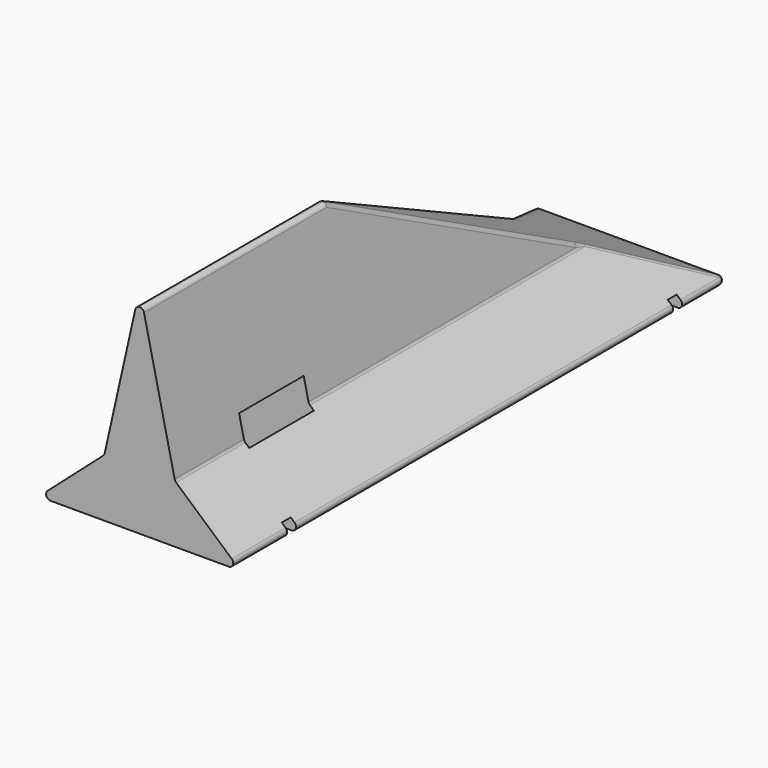
from build123d import *

# Parameters (mm, degrees)
F1_DEPTH = 28.575
F3_DEPTH = 22.86
F5_DEPTH = 177.8
F6_R     = 1.27


with BuildPart() as f1:
    # F0 (on Right) → F1 (new body, symmetric)
    with BuildSketch(Plane.YZ):
        Polygon((-57.9421781003, 88.9), (-57.9421781003, 0), (-38.8921781003, 0), (-38.8921781003, 3.175), (-35.7171781003, 3.175), (-35.7171781003, 0), (97.6328218997, 0), (97.6328218997, 3.175), (100.8078218997, 3.175), (100.8078218997, 0), (119.8578218997, 0), align=None)
    extrude(amount=F1_DEPTH, both=True)

    # F2 (on face) → F3 (cut)
    with BuildSketch(Plane(origin=(0, 0, 0), x_dir=(1, 0, 0), z_dir=(0, 0, -1))):
        Polygon((11.43, 33.4499907649), (0, 33.4499907649), (-11.43, 33.4499907649), (-11.43, 10.5899907649), (0, 10.5899907649), (11.43, 10.5899907649), align=None)
    extrude(amount=-F3_DEPTH, mode=Mode.SUBTRACT)

    # F4 (on face) → F5 (intersect)
    with BuildSketch(Plane.XZ.offset(57.9421781003)):
        Polygon((-9.9975576818, 16.3837641232), (-28.575, 0), (28.575, 0), (9.9975576818, 16.3837641232), (0, 60.9972961555), align=None)
    extrude(amount=-F5_DEPTH, mode=Mode.INTERSECT)

    # F6
    f6_edges = [f1.edges().sort_by_distance(p)[0] for p in [
        (0, 119.857822, 0),
        (4.998779, 42.476762, 38.69053),
        (-4.998779, 42.476762, 38.69053),
        (19.286279, 103.474058, 8.191882),
        (-19.286279, 103.474058, 8.191882),
        (0, -30.039474, 60.997296),
        (9.997558, 38.250151, 16.383764),
        (28.575, 30.957822, 0),
        (28.575, -48.417178, 0),
        (28.575, 110.332822, 0),
        (-28.575, 110.332822, 0),
        (-28.575, 30.957822, 0),
        (-28.575, -48.417178, 0),
        (-9.997558, 38.250151, 16.383764),
        (-9.997558, -45.696084, 16.383764),
        (9.997558, -45.696084, 16.383764),
    ]]
    fillet(f6_edges, radius=F6_R)


solid = f1.part
